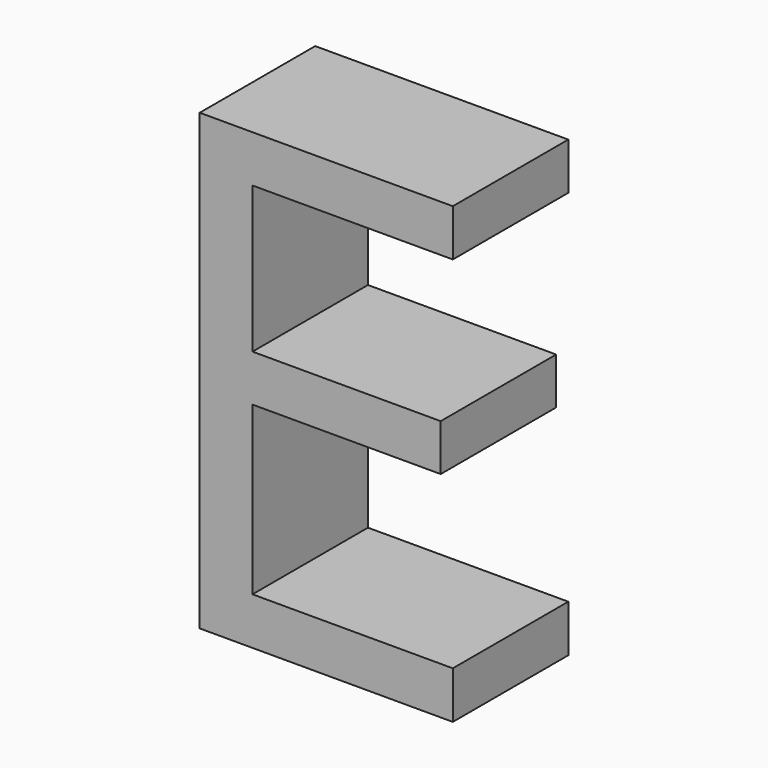
from build123d import *

# Parameters (mm, degrees)
F0_TEXT_SIZE = 110.1586553786
F1_DEPTH     = 25


# Not quite as in the source:
# - Text() gives the source's letters only with a copy of the font that has no kerning and outlines rounded to 1/6400 em; it was checked with that copy


with BuildPart() as f1:
    # F0 (on Front) → F1 (new body)
    with BuildSketch(Plane.XZ):
        with Locations((-56.8257458508, -35.7092022896)):
            Text('E', F0_TEXT_SIZE, font='Open Sans', text_align=(TextAlign.LEFT, TextAlign.BOTTOM))
    extrude(amount=F1_DEPTH)


solid = f1.part
